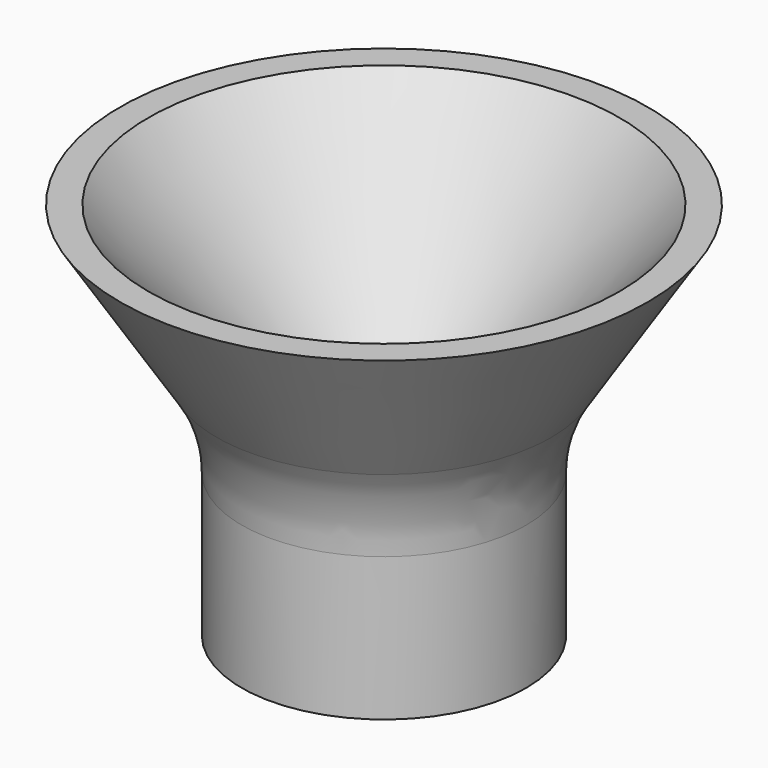
from build123d import *

# Parameters (mm, degrees)
F0_R     = 9
F0_R_2   = 7.6
F3_DEPTH = 12
F5_R     = 10


# Not quite as in the source:
# - a feature names something its author has since deleted; it is built from what else it names


with BuildPart() as f3:
    # F0 (on Top) → F3 (new body)
    with BuildSketch(Plane.XY):
        Circle(F0_R)
        Circle(F0_R_2, mode=Mode.SUBTRACT)
    extrude(amount=F3_DEPTH)

    # F1 (on Front) → F4 (revolve)
    with BuildSketch(Plane.XZ):
        Polygon((14.9, 24), (4.5, 12), (9, 12), (16.7, 24), align=None)
    revolve(axis=Axis((0, 0, -6.017471198), (0, 0, -1)))

    # F5
    f5_edges = [f3.edges().sort_by_distance(p)[0] for p in [
        (-9, 0, 12),
    ]]
    fillet(f5_edges, radius=F5_R)


solid = f3.part
